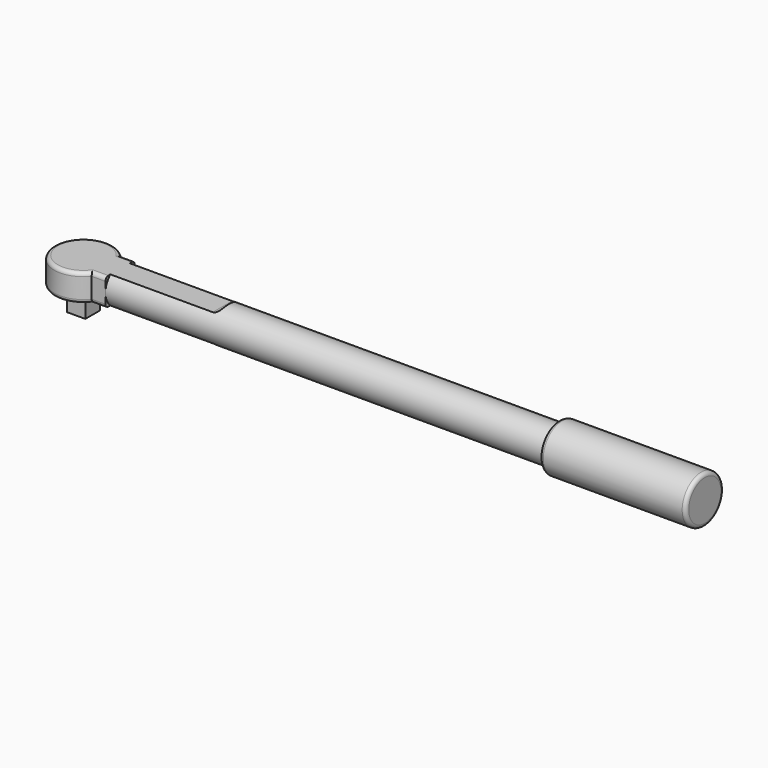
from build123d import *

# Parameters (mm, degrees)
F0_R        = 12.7
F1_DEPTH    = 406.4
F2_R        = 16.51
F3_DEPTH    = 101.6
F5_DEPTH    = 9.525
F6_W        = 76.2
F6_H        = 3.175
F7_DEPTH    = 12.7
F8_T4_DEPTH = 42.2005208253
F8_S5_R     = 12.7
F8_T6_DEPTH = 23
F9_T4_DEPTH = 42.2005208253
F9_S5_R     = 12.7
F9_T6_DEPTH = 23
F10_R       = 2.54
F11_W       = 12.7
F11_H       = 12.7
F12_DEPTH   = 15.24


# Not quite as in the source:
# - a fillet or chamfer that OpenCascade refuses, or shapes differently, is made with other operations: its cross-section is extruded or revolved along the edge and cut away or added


with BuildPart() as f1:
    # F0 (on Right) → F1 (new body)
    with BuildSketch(Plane.YZ):
        Circle(F0_R)
    extrude(amount=F1_DEPTH)

    # F2 (on face) → F3 (join)
    with BuildSketch(Plane.YZ.offset(406.4)):
        Circle(F2_R)
    extrude(amount=-F3_DEPTH)

    # F4 (on Top) → F5 (join, symmetric)
    with BuildSketch(Plane.XY):
        with BuildLine():
            Line((0, 12.7), (-9.5377050841, 12.7))
            ThreePointArc((-9.5377050841, 12.7), (-45.72, 0), (-9.5377050841, -12.7))
            Line((-9.5377050841, -12.7), (0, -12.7))
            Line((0, -12.7), (0, 12.7))
        make_face()
    extrude(amount=F5_DEPTH, both=True)

    # F6 (on Front) → F7 (cut, symmetric)
    with BuildSketch(Plane.XZ):
        with Locations((38.1, 11.1125)):
            Rectangle(F6_W, F6_H)
        with Locations((38.1, -11.1125)):
            Rectangle(F6_W, F6_H)
    extrude(amount=F7_DEPTH, both=True, mode=Mode.SUBTRACT)

    # F8: fillet of radius 5.08 on 1 edges, made by hand


with BuildPart() as f8_tool2:
    # F8_s3 → F8_t4 (new body)
    with BuildSketch(Plane.XZ.offset(-21.1002604126)):
        with BuildLine():
            ThreePointArc((76.2, 14.605), (74.7121024484, 11.0128975516), (71.12, 9.525))
            Line((71.12, 9.525), (76.2, 9.525))
            Line((76.2, 9.525), (76.2, 14.605))
        make_face()
    extrude(amount=F8_T4_DEPTH)

    # F8_s5 → F8_t6 (intersect, symmetric)
    with BuildSketch(Plane.YZ.offset(73.7)):
        Circle(F8_S5_R)
    extrude(amount=F8_T6_DEPTH, both=True, mode=Mode.INTERSECT)


with BuildPart() as f1_1:
    add(f1.part)

    # F8_t1: union F8_tool2
    add(f8_tool2.part)

    # F9: fillet of radius 5.08 on 1 edges, made by hand


with BuildPart() as f9_tool2:
    # F9_s3 → F9_t4 (new body)
    with BuildSketch(Plane.XZ.offset(21.1002604126)):
        with BuildLine():
            ThreePointArc((71.12, -9.525), (74.7121024484, -11.0128975516), (76.2, -14.605))
            Line((76.2, -14.605), (76.2, -9.525))
            Line((76.2, -9.525), (71.12, -9.525))
        make_face()
    extrude(amount=-F9_T4_DEPTH)

    # F9_s5 → F9_t6 (intersect, symmetric)
    with BuildSketch(Plane.YZ.offset(73.7)):
        Circle(F9_S5_R)
    extrude(amount=F9_T6_DEPTH, both=True, mode=Mode.INTERSECT)


with BuildPart() as f1_2:
    add(f1_1.part)

    # F9_t1: union F9_tool2
    add(f9_tool2.part)

    # F10
    f10_edges = [f1_2.edges().sort_by_distance(p)[0] for p in [
        (-45.72, 0, -9.525),
        (-45.72, 0, 9.525),
        (-4.768853, -12.7, -9.525),
        (-4.768853, -12.7, 9.525),
        (-4.768853, 12.7, -9.525),
        (-4.768853, 12.7, 9.525),
        (406.4, -16.51, 0),
        (304.8, -16.51, 0),
    ]]
    fillet(f10_edges, radius=F10_R)

    # F11 (on face) → F12 (join)
    with BuildSketch(Plane(origin=(0, 0, -9.525), x_dir=(1, 0, 0), z_dir=(0, 0, -1))):
        with Locations((-25.4, 0)):
            Rectangle(F11_W, F11_H)
    extrude(amount=F12_DEPTH)


solid = f1_2.part
